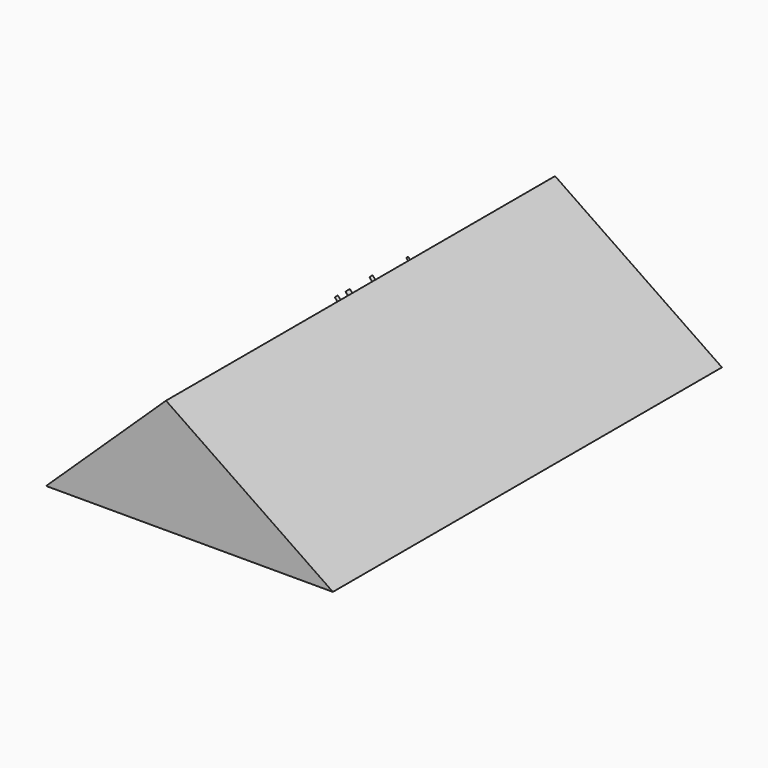
from build123d import *

# Parameters (mm, degrees)
F1_DEPTH  = 21336
F2_R      = 38.1
F3_DEPTH  = 254
F4_R      = 38.1
F5_DEPTH  = 254
F6_R      = 38.1
F7_DEPTH  = 254
F8_R      = 63.5
F9_DEPTH  = 254
F10_R     = 63.5
F11_DEPTH = 254
F12_R     = 88.9
F13_DEPTH = 254
F15_DEPTH = 254


with BuildPart() as f1:
    # F0 (on Front) → F1 (new body)
    with BuildSketch(Plane.XZ):
        Polygon((0, 5007.909211275), (-5262.3523914336, 0), (7321.0311030403, 0), align=None)
    extrude(amount=F1_DEPTH)

    # F2 (on face) → F3 (join)
    with BuildSketch(Plane(origin=(-2500.8826949727, 0, 2627.9482065997), x_dir=(0.7244028951, 0, 0.689376853), z_dir=(-0.689376853, 0, 0.7244028951))):
        with Locations((-433.8633075859, -2082.8)):
            Circle(F2_R)
    extrude(amount=F3_DEPTH)

    # F4 (on face) → F5 (join)
    with BuildSketch(Plane(origin=(-2500.8826949727, 0, 2627.9482065997), x_dir=(0.7244028951, 0, 0.689376853), z_dir=(-0.689376853, 0, 0.7244028951))):
        with Locations((-3329.4633075859, -11455.4)):
            Circle(F4_R)
    extrude(amount=F5_DEPTH)

    # F6 (on face) → F7 (join)
    with BuildSketch(Plane(origin=(-2500.8826949727, 0, 2627.9482065997), x_dir=(0.7244028951, 0, 0.689376853), z_dir=(-0.689376853, 0, 0.7244028951))):
        with Locations((1445.7366924141, -6070.6)):
            Circle(F6_R)
    extrude(amount=F7_DEPTH)

    # F8 (on face) → F9 (join)
    with BuildSketch(Plane(origin=(-2500.8826949727, 0, 2627.9482065997), x_dir=(0.7244028951, 0, 0.689376853), z_dir=(-0.689376853, 0, 0.7244028951))):
        with Locations((2309.3366924141, -8839.2)):
            Circle(F8_R)
    extrude(amount=F9_DEPTH)

    # F10 (on face) → F11 (join)
    with BuildSketch(Plane(origin=(-2500.8826949727, 0, 2627.9482065997), x_dir=(0.7244028951, 0, 0.689376853), z_dir=(-0.689376853, 0, 0.7244028951))):
        with Locations((2309.3366924141, -10744.2)):
            Circle(F10_R)
    extrude(amount=F11_DEPTH)

    # F12 (on face) → F13 (join)
    with BuildSketch(Plane(origin=(-2500.8826949727, 0, 2627.9482065997), x_dir=(0.7244028951, 0, 0.689376853), z_dir=(-0.689376853, 0, 0.7244028951))):
        with Locations((2017.2366924141, -9855.2)):
            Circle(F12_R)
    extrude(amount=F13_DEPTH)

    # F14 (on face) → F15 (join)
    with BuildSketch(Plane(origin=(-2500.8826949727, 0, 2627.9482065997), x_dir=(0.7244028951, 0, 0.689376853), z_dir=(-0.689376853, 0, 0.7244028951))):
        Polygon((-1780.0633075859, -4724.4), (-3812.0633075859, -3048), (-3812.0633075859, -6400.8), align=None)
    extrude(amount=F15_DEPTH)


solid = f1.part
